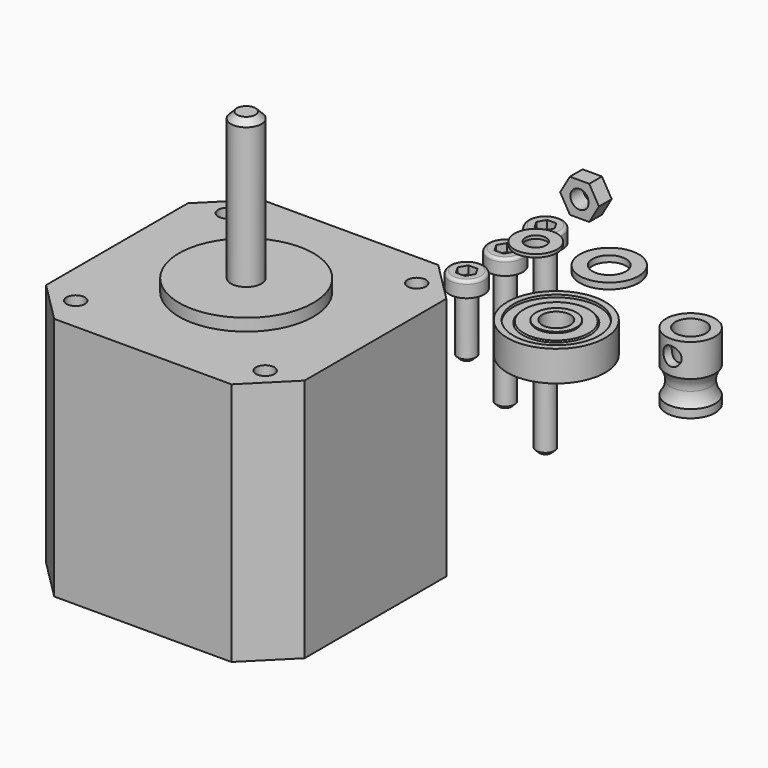
from build123d import *

# Parameters (mm, degrees)
F0_R       = 1.5
F2_DEPTH   = 25
F4_R       = 11
F4_R_2     = 2.5
F5_DEPTH   = 2
F6_DEPTH   = 26
F7_DEPTH   = 40
F8_D       = 3
F8_DEPTH   = 4.5
F8_TIP     = 0.9012909285
F9_SIZE    = 1
F0_W       = 1.81
F0_H       = 0.5
F0_W_2     = 1.5
F0_H_2     = 10
F13_DEPTH  = 1.3
F15_DEPTH  = 20
F0_W_3     = 2.08
F0_H_3     = 1
F18_DEPTH  = 10
F19_SIZE   = 0.5
F19_2_SIZE = 0.5
F19_3_SIZE = 0.5
F20_DEPTH  = 2.6


with BuildPart() as f1:
    # F0 (on Front) → F1 (revolve)
    with BuildSketch(Plane.XZ):
        with BuildLine():
            Line((-23.1557391211, 19.3900806742), (-24.6557391211, 19.3900806742))
            Line((-24.6557391211, 19.3900806742), (-24.6557391211, 14.0551441836))
            ThreePointArc((-24.6557391211, 14.0551441836), (-24.0985499823, 13.0357245979), (-23.9057391211, 11.8900806742))
            ThreePointArc((-23.9057391211, 11.8900806742), (-24.0985499823, 10.7444367504), (-24.6557391211, 9.7250171647))
            Line((-24.6557391211, 9.7250171647), (-24.6557391211, 8.3900806742))
            Line((-24.6557391211, 8.3900806742), (-23.1557391211, 8.3900806742))
            Line((-23.1557391211, 8.3900806742), (-23.1557391211, 19.3900806742))
        make_face()
    revolve(axis=Axis((-20.6557391211, 0, 13.8900806742), (0, 0, -1)))

    # F0 (on Front) → F2 (cut)
    with BuildSketch(Plane.XZ):
        with Locations((-20.6557391211, 16.8900806742)):
            Circle(F0_R)
    extrude(amount=F2_DEPTH, mode=Mode.SUBTRACT)


with BuildPart() as f3:
    # F0 (on Front) → F3 (revolve)
    with BuildSketch(Plane.XZ):
        Polygon((-49.6386482716, 13.3454260603), (-50.6386482716, 13.3454260603), (-50.6386482716, 8.3454260603), (-49.6386482716, 8.3454260603), (-49.6386482716, 8.7454260603), (-48.1386482716, 8.7454260603), (-47.9386482716, 8.5454260603), (-45.9386482716, 8.5454260603), (-45.9386482716, 8.3454260603), (-44.9386482716, 8.3454260603), (-44.9386482716, 13.3454260603), (-45.9386482716, 13.3454260603), (-45.9386482716, 13.1454260603), (-47.9386482716, 13.1454260603), (-48.1386482716, 12.9454260603), (-49.6386482716, 12.9454260603), align=None)
    revolve(axis=Axis((-42.6386482716, 0, 10.8454260603), (0, 0, -1)))


with BuildPart() as f5:
    # F4 (on Top) → F5 (new body)
    with BuildSketch(Plane.XY):
        with Locations((-94.4311614871, 1.3196146563)):
            Circle(F4_R)
        with Locations((-94.4311614871, 1.3196146563)):
            Circle(F4_R_2, mode=Mode.SUBTRACT)
        with Locations((-94.4311614871, 1.3196146563)):
            Circle(F4_R_2)
    extrude(amount=F5_DEPTH)

    # F4 (on Top) → F6 (join)
    with BuildSketch(Plane.XY):
        with Locations((-94.4311614871, 1.3196146563)):
            Circle(F4_R_2)
    extrude(amount=F6_DEPTH)

    # F4 (on Top) → F7 (join)
    with BuildSketch(Plane.XY):
        Polygon((-108.9311614871, 22.4696146563), (-115.5811614871, 15.8196146563), (-115.5811614871, -13.1803853437), (-108.9311614871, -19.8303853437), (-79.9311614871, -19.8303853437), (-73.2811614871, -13.1803853437), (-73.2811614871, 15.8196146563), (-79.9311614871, 22.4696146563), align=None)
        with Locations((-94.4311614871, 1.3196146563)):
            Circle(F4_R, mode=Mode.SUBTRACT)
        with Locations((-94.4311614871, 1.3196146563)):
            Circle(F4_R)
        with Locations((-94.4311614871, 1.3196146563)):
            Circle(F4_R_2, mode=Mode.SUBTRACT)
        with Locations((-94.4311614871, 1.3196146563)):
            Circle(F4_R_2)
    extrude(amount=-F7_DEPTH)

    # F8
    with Locations(Plane.XY):
        with Locations((-78.9311614871, 16.8196146563), (-78.9311614871, -14.1803853437), (-109.9311614871, -14.1803853437), (-109.9311614871, 16.8196146563)):
            Hole(F8_D / 2, depth=F8_DEPTH)
            with Locations((0, 0, -(F8_DEPTH + F8_TIP / 2))):  # 118° drill point
                Cone(0, F8_D / 2, F8_TIP, mode=Mode.SUBTRACT)

    # F9
    f9_edges = [f5.edges().sort_by_distance(p)[0] for p in [
        (-96.931161, 1.319615, 26),
    ]]
    chamfer(f9_edges, length=F9_SIZE)


with BuildPart() as f10:
    # F0 (on Front) → F10 (revolve)
    with BuildSketch(Plane.XZ):
        with Locations((-48.5946421039, 23.3027455807)):
            Rectangle(F0_W, F0_H)
    revolve(axis=Axis((-45.9996421039, 0, 23.3027455807), (0, 0, -1)))


with BuildPart() as f11:
    # F0 (on Front) → F11 (revolve)
    with BuildSketch(Plane.XZ):
        with BuildLine():
            ThreePointArc((-59.6368863547, 15.6719975471), (-59.9904397453, 15.5255509377), (-60.1368863547, 15.1719975471))
            Line((-60.1368863547, 15.1719975471), (-60.1368863547, 13.1719975471))
            Line((-60.1368863547, 13.1719975471), (-58.7968863547, 13.1719975471))
            Line((-58.7968863547, 13.1719975471), (-57.2968863547, 13.1719975471))
            Line((-57.2968863547, 13.1719975471), (-57.2968863547, 15.6719975471))
            Line((-57.2968863547, 15.6719975471), (-59.6368863547, 15.6719975471))
        make_face()
        with Locations((-58.0468863547, 8.1719975471)):
            Rectangle(F0_W_2, F0_H_2)
    revolve(axis=Axis((-57.2968863547, 0, 8.1719975471), (0, 0, -1)))

    # F12 (on face) → F13 (cut)
    with BuildSketch(Plane.XY.offset(15.6719975471)):
        Polygon((-56.5521045074, 1.29), (-58.0416682019, 1.29), (-58.7864500492, 0), (-58.0416682019, -1.29), (-56.5521045074, -1.29), (-55.8073226602, 0), align=None)
    extrude(amount=-F13_DEPTH, mode=Mode.SUBTRACT)


with BuildPart() as f14_1:
    # F14: copy of F11
    add(f11.part.moved(Location((0, 16.1, 0))))

    # F15 (add): a face of the model
    f15_faces = [f14_1.faces().sort_by_distance(p)[0] for p in [
        (-57.2968863547, 16.1, 3.1719975471),
    ]]
    extrude(f15_faces, amount=F15_DEPTH)

    # F19#2
    f19_2_edges = [f14_1.edges().sort_by_distance(p)[0] for p in [
        (-55.796886, 16.1, -16.828002),
    ]]
    chamfer(f19_2_edges, length=F19_2_SIZE)


with BuildPart() as f16:
    # F0 (on Front) → F16 (revolve)
    with BuildSketch(Plane.XZ):
        with Locations((-37.7473910367, 23.5527455807)):
            Rectangle(F0_W_3, F0_H_3)
    revolve(axis=Axis((-33.9673910367, 0, 23.5527455807), (0, 0, 1)))


with BuildPart() as f17_1:
    # F17: copy of F11
    add(f11.part.moved(Location((0, 7.9, 0))))

    # F18 (add): a face of the model
    f18_faces = [f17_1.faces().sort_by_distance(p)[0] for p in [
        (-57.2968863547, 7.9, 3.1719975471),
    ]]
    extrude(f18_faces, amount=F18_DEPTH)

    # F19#3
    f19_3_edges = [f17_1.edges().sort_by_distance(p)[0] for p in [
        (-55.796886, 7.9, -6.828002),
    ]]
    chamfer(f19_3_edges, length=F19_3_SIZE)


with BuildPart() as f11_1:
    add(f11.part)

    # F19
    f19_edges = [f11_1.edges().sort_by_distance(p)[0] for p in [
        (-55.796886, 0, 3.171998),
    ]]
    chamfer(f19_edges, length=F19_SIZE)


with BuildPart() as f20:
    # F0 (on Front) → F20 (new body)
    with BuildSketch(Plane.XZ):
        Polygon((-38.338067113, 30.9423487484), (-35.1626406325, 30.9423487484), (-33.5749273922, 33.6923487484), (-35.1626406325, 36.4423487484), (-38.338067113, 36.4423487484), (-39.9257803533, 33.6923487484), align=None)
        with Locations((-36.7503538728, 33.6923487484)):
            Circle(F0_R, mode=Mode.SUBTRACT)
    extrude(amount=F20_DEPTH)


solid = Compound([f1.part, f3.part, f5.part, f10.part, f14_1.part, f16.part, f17_1.part, f11_1.part, f20.part])
